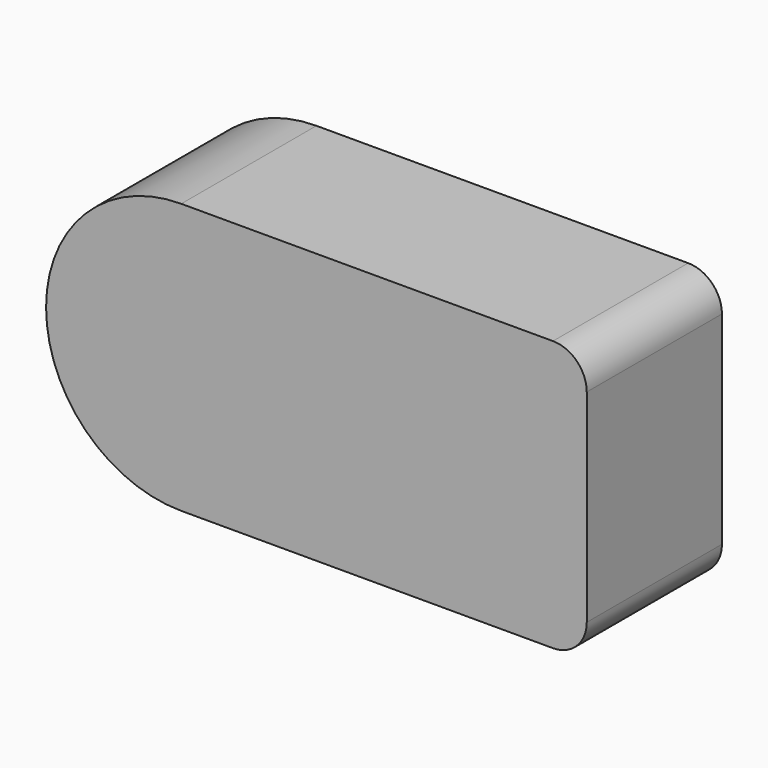
from build123d import *

# Parameters (mm, degrees)
F0_W     = 80
F0_H     = 40
F1_DEPTH = 25
F2_R     = 20
F3_R     = 19.99999
F4_R     = 5


# Not quite as in the source:
# - a fillet or chamfer is up to 0.001 mm smaller than in the source, because OpenCascade refuses the exact size


with BuildPart() as f1:
    # F0 (on Front) → F1 (new body)
    with BuildSketch(Plane.XZ):
        with Locations((40, 20)):
            Rectangle(F0_W, F0_H)
    extrude(amount=F1_DEPTH)

    # F2
    f2_edges = [f1.edges().sort_by_distance(p)[0] for p in [
        (0, -12.5, 40),
    ]]
    fillet(f2_edges, radius=F2_R)

    # F3 (radius 20 in the source; OpenCascade refuses exactly that, so slightly less here)
    f3_edges = [f1.edges().sort_by_distance(p)[0] for p in [
        (0, -12.5, 0),
    ]]
    fillet(f3_edges, radius=F3_R)

    # F4
    f4_edges = [f1.edges().sort_by_distance(p)[0] for p in [
        (80, -12.5, 40),
        (80, -12.5, 0),
    ]]
    fillet(f4_edges, radius=F4_R)


solid = f1.part
